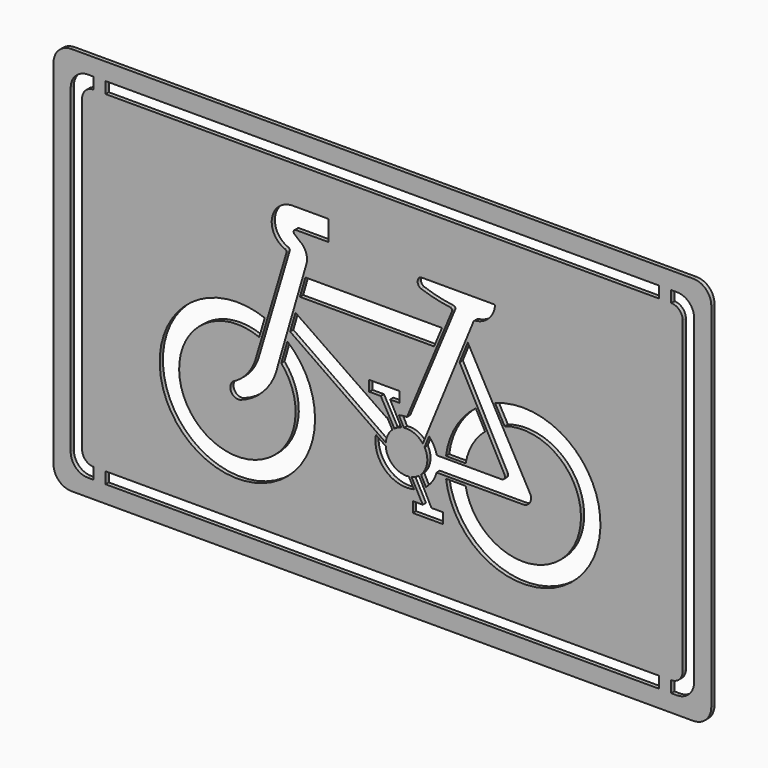
from build123d import *

# Parameters (mm, degrees)
F0_W     = 412.447963
F0_H     = 8.529411
F0_H_2   = 8.529412
F1_DEPTH = 3


# Not quite as in the source:
# - ends of sketch curves that miss each other by under 0.0002 mm in the source are joined


with BuildPart() as f1:
    # F0 (on Front) → F1 (new body)
    with BuildSketch(Plane.XZ):
        with BuildLine():
            Line((-245, 131.615385), (-245, -131.615384))
            ThreePointArc((-245, -131.615384), (-241.0797377372, -141.0797367372), (-231.615385, -145))
            Line((-231.615385, -145), (231.615384, -145))
            ThreePointArc((231.615384, -145), (241.0797367372, -141.0797367372), (245, -131.615384))
            Line((245, -131.615384), (245, 131.615385))
            ThreePointArc((245, 131.615385), (241.0797367372, 141.0797377372), (231.615384, 145.000001))
            Line((231.615384, 145.000001), (-231.615385, 145))
            ThreePointArc((-231.615385, 145), (-241.0797377372, 141.0797377372), (-245, 131.615385))
        make_face()
        with BuildLine():
            ThreePointArc((-223.67647, -115.147058), (-221.1782633576, -121.1782623576), (-215.147059, -123.676469))
            Line((-215.147059, -123.676469), (-215.147059, -132.205882))
            Line((-215.147059, -132.205882), (-219.411765, -132.205882))
            ThreePointArc((-219.411765, -132.205882), (-228.4585725971, -128.4585725971), (-232.205883, -119.411765))
            Line((-232.205883, -119.411765), (-232.205883, 119.411764))
            ThreePointArc((-232.205883, 119.411764), (-228.4585725971, 128.4585715971), (-219.411765, 132.205882))
            Line((-219.411765, 132.205882), (-215.147059, 132.205883))
            Line((-215.147059, 132.205883), (-215.147059, 123.676471))
            ThreePointArc((-215.147059, 123.676471), (-221.1782633576, 121.1782633576), (-223.67647, 115.147059))
            Line((-223.67647, 115.147059), (-223.67647, -115.147058))
        make_face(mode=Mode.SUBTRACT)
        with BuildLine():
            ThreePointArc((-70.7599172527, 5.5663826998), (-137.2958198093, -88.6390266704), (-87.6127799718, 15.4440220749))
            Line((-87.6127799718, 15.4440220749), (-91.766694, 1.50065))
            ThreePointArc((-91.766694, 1.50065), (-133.2066284732, -74.0292729296), (-75.3272882753, -10.2168972398))
            Line((-75.3272882753, -10.2168972398), (-70.7599172527, 5.5663826998))
        make_face(mode=Mode.SUBTRACT)
        with BuildLine():
            Line((-68.723593, 12.582627), (-64.743288, 26.326147))
            Line((-64.743288, 26.326147), (3.159571, -20.475886))
            ThreePointArc((3.159571, -20.475886), (3.3683994767, -20.3043898267), (3.5792137936, -20.1353407395))
            Line((3.5792137936, -20.1353407395), (7.411744, -26.95528))
            ThreePointArc((7.411744, -26.95528), (4.0249471652, -31.5409295129), (2.5258681402, -37.0410509302))
            Line((2.5258681402, -37.0410509302), (-68.723593, 12.582627))
        make_face(mode=Mode.SUBTRACT)
        with Locations((-5e-07, -127.9411765)):
            Rectangle(F0_W, F0_H, mode=Mode.SUBTRACT)
        with BuildLine():
            Line((22.72508, -68.805566), (30.090636, -68.805566))
            Line((30.090636, -68.805566), (21.674726, -53.339399))
            ThreePointArc((21.674726, -53.339399), (24.591046355, -52.3025256725), (27.243072314, -50.7066594202))
            Line((27.243072314, -50.7066594202), (36.565765, -68.805566))
            Line((36.565765, -68.805566), (45.281341, -68.805566))
            Line((45.281341, -68.805566), (45.281341, -76.614964))
            Line((45.281341, -76.614964), (22.72508, -76.614964))
            Line((22.72508, -76.614964), (22.72508, -68.805566))
        make_face(mode=Mode.SUBTRACT)
        with BuildLine():
            Line((-4.847605, -34.261624), (2.51358, -39.388528))
            ThreePointArc((2.51358, -39.388528), (8.0448119147, -50.1939653909), (19.6676101132, -53.6957600257))
            Line((19.6676101132, -53.6957600257), (23.527377, -60.788967))
            ThreePointArc((23.527377, -60.788967), (2.1451797481, -55.2211156409), (-4.847605, -34.261624))
        make_face(mode=Mode.SUBTRACT)
        with BuildLine():
            ThreePointArc((83.96580189, 15.3881272867), (154.3064474066, -68.0805916135), (47.3881182197, -46.096407971))
            Line((47.3881182197, -46.096407971), (62.056469, -46.096408))
            ThreePointArc((62.056469, -46.096408), (141.8170821306, -60.7137946065), (91.0686279767, 2.5318990705))
            Line((91.0686279767, 2.5318990705), (83.96580189, 15.3881272867))
        make_face(mode=Mode.SUBTRACT)
        with BuildLine():
            Line((8.930442, -25.711427), (-1.213114, -7.6611))
            Line((-1.213114, -7.6611), (-9.807377, -7.6611))
            Line((-9.807377, -7.6611), (-9.807377, 0.1483))
            Line((-9.807377, 0.1483), (12.748884, 0.1483))
            Line((12.748884, 0.1483), (12.748884, -7.6611))
            Line((12.748884, -7.6611), (5.767885, -7.6611))
            Line((5.767885, -7.6611), (14.045243, -23.30707))
            ThreePointArc((14.045243, -23.30707), (11.3772825006, -24.2740536292), (8.930442, -25.711427))
        make_face(mode=Mode.SUBTRACT)
        with BuildLine():
            ThreePointArc((47.3586275037, -31.2217609366), (54.5791913728, -9.7531888086), (69.4990666913, 7.2889194025))
            Line((69.4990666913, 7.2889194025), (76.442916, -5.74499))
            ThreePointArc((76.442916, -5.74499), (67.0095000702, -17.2261004781), (62.0168330844, -31.2217610145))
            Line((62.0168330844, -31.2217610145), (47.3586275037, -31.2217609366))
        make_face(mode=Mode.SUBTRACT)
        with BuildLine():
            Line((90.984376, -29.244421), (57.508949, 33.590423))
            Line((57.508949, 33.590423), (63.619612, 48.524677))
            Line((63.619612, 48.524677), (110.016211, -35.453915))
            ThreePointArc((110.016211, -35.453915), (109.9324845309, -41.3751059281), (104.790172, -44.311794))
            Line((104.790172, -44.311794), (40.343874, -44.311793))
            ThreePointArc((40.343874, -44.311793), (37.3331086152, -51.0181961304), (32.3730594707, -56.443918593))
            Line((32.3730594707, -56.443918593), (28.754286, -49.418498))
            ThreePointArc((28.754286, -49.418498), (33.3103193803, -40.4589080248), (31.409337593, -30.5888542334))
            Line((31.409337593, -30.5888542334), (34.77995, -22.351191))
            ThreePointArc((34.77995, -22.351191), (38.3615541693, -27.2968191094), (40.5267526716, -33.006376077))
            Line((40.5267526716, -33.006376077), (88.726046, -33.006377))
            ThreePointArc((88.726046, -33.006377), (90.9199219225, -31.7645528859), (90.984376, -29.244421))
        make_face(mode=Mode.SUBTRACT)
        with BuildLine():
            Line((219.411764, -132.205882), (215.147059, -132.205882))
            Line((215.147059, -132.205882), (215.147059, -123.676471))
            ThreePointArc((215.147059, -123.676471), (221.1782633576, -121.1782623576), (223.67647, -115.147058))
            Line((223.67647, -115.147058), (223.67647, 115.147059))
            ThreePointArc((223.67647, 115.147059), (221.1782633576, 121.1782633576), (215.147059, 123.67647))
            Line((215.147059, 123.67647), (215.147059, 132.205883))
            Line((215.147059, 132.205883), (219.411764, 132.205882))
            ThreePointArc((219.411764, 132.205882), (228.4585715971, 128.4585715971), (232.205882, 119.411764))
            Line((232.205882, 119.411764), (232.205881, -119.411765))
            ThreePointArc((232.205881, -119.411765), (228.4585715971, -128.4585725971), (219.411764, -132.205882))
        make_face(mode=Mode.SUBTRACT)
        with BuildLine():
            ThreePointArc((-72.4661841519, 65.5207366103), (-82.1538966479, 83.216021136), (-66.4060260229, 95.8247260113))
            Line((-66.4060260229, 95.8247260113), (-40.035993, 95.824726))
            Line((-40.035993, 95.824726), (-40.035993, 80.630917))
            Line((-40.035993, 80.630917), (-64.424786, 80.630917))
            ThreePointArc((-64.424786, 80.630917), (-66.0282591874, 79.5071913113), (-65.5192035969, 77.616491482))
            Line((-65.5192035969, 77.616491482), (-59.43939, 72.531557))
            ThreePointArc((-59.43939, 72.531557), (-56.3975970197, 66.4763179948), (-56.9296708586, 59.7209263141))
            Line((-56.9296708586, 59.7209263141), (-77.850161, -12.515038))
            ThreePointArc((-77.850161, -12.515038), (-87.3559409811, -31.7459411903), (-105.0135430166, -43.9277549547))
            ThreePointArc((-105.0135430166, -43.9277549547), (-112.4545221205, -41.478665578), (-111.0494858176, -33.7720412284))
            ThreePointArc((-111.0494858176, -33.7720412284), (-101.1018664771, -25.9057272999), (-94.7919815143, -14.9048461665))
            Line((-94.7919815143, -14.9048461665), (-71.450754, 63.444245))
            ThreePointArc((-71.450754, 63.444245), (-71.5531660844, 64.6806886283), (-72.4661841519, 65.5207366103))
        make_face(mode=Mode.SUBTRACT)
        Polygon((-61.428563, 37.771498), (-57.350449, 51.85274), (44.398561, 51.85274), (38.504827, 37.771498), align=None, mode=Mode.SUBTRACT)
        with BuildLine():
            ThreePointArc((12.2794031528, -15.8349486032), (15.2656197234, -15.2838363253), (18.2982629962, -15.1279872662))
            Line((18.2982629962, -15.1279872662), (51.823582, 64.970319))
            ThreePointArc((51.823582, 64.970319), (51.7665690353, 66.512857989), (50.4881340177, 67.3778901407))
            ThreePointArc((50.4881340177, 67.3778901407), (39.4345578147, 69.3755880777), (28.6570272111, 72.5405805985))
            ThreePointArc((28.6570272111, 72.5405805985), (26.2908771018, 75.8079169957), (27.8157723755, 79.5427327786))
            ThreePointArc((27.8157723755, 79.5427327786), (28.3174115009, 79.8213352122), (28.883051, 79.917843))
            Line((28.883051, 79.917843), (83.068308, 79.917844))
            ThreePointArc((83.068308, 79.917844), (83.7102572475, 79.6265153128), (83.9136824011, 78.9515420803))
            ThreePointArc((83.9136824011, 78.9515420803), (79.0432795601, 69.2443269594), (69.2278859862, 64.5957881246))
            ThreePointArc((69.2278859862, 64.5957881246), (68.3724892885, 64.249714451), (67.8224577861, 63.5088130817))
            Line((67.8224577861, 63.5088130817), (30.106815, -28.666942))
            ThreePointArc((30.106815, -28.666942), (23.8211455462, -23.950033286), (16.0297460076, -22.92389506))
            Line((16.0297460076, -22.92389506), (12.2794031528, -15.8349486032))
        make_face(mode=Mode.SUBTRACT)
        with Locations((-5e-07, 127.941177)):
            Rectangle(F0_W, F0_H_2, mode=Mode.SUBTRACT)
    extrude(amount=F1_DEPTH)


solid = f1.part
